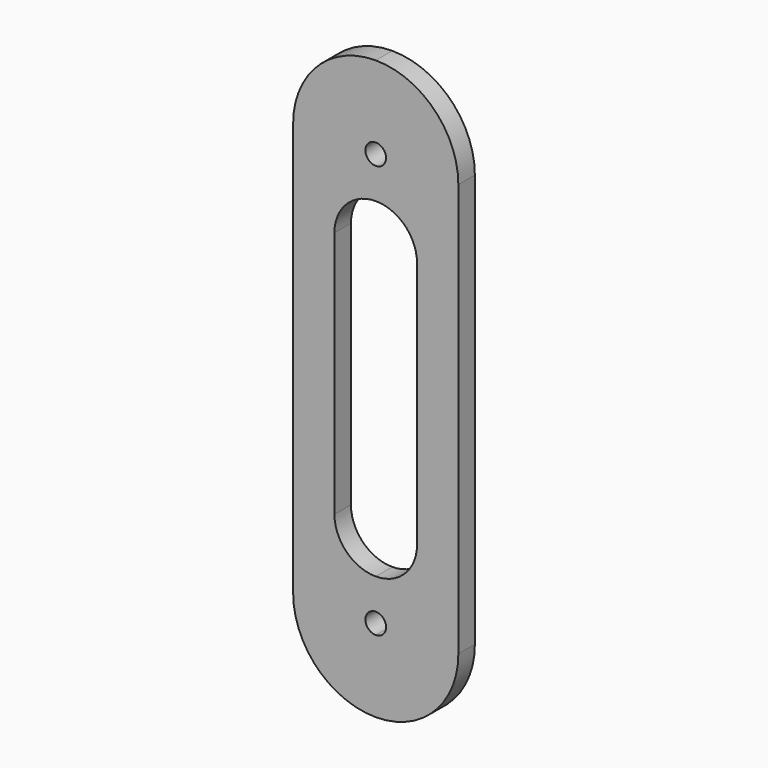
from build123d import *

# Parameters (mm, degrees)
F1_DEPTH = 1.5875


with BuildPart() as f1:
    # F0 (on Front) → F1 (new body, symmetric)
    with BuildSketch(Plane.XZ):
        with BuildLine():
            Line((0, 76.2), (0, 12.7))
            ThreePointArc((0, 12.7), (3.719744, 3.719744), (12.7, 0))
            Line((12.7, 0), (12.7, 11.1125))
            ThreePointArc((12.7, 11.1125), (11.1125, 12.7), (12.7, 14.2875))
            Line((12.7, 14.2875), (12.7, 19.05))
            ThreePointArc((12.7, 19.05), (8.209872, 20.909872), (6.35, 25.4))
            Line((6.35, 25.4), (6.35, 63.5))
            ThreePointArc((6.35, 63.5), (8.209872, 67.990128), (12.7, 69.85))
            Line((12.7, 69.85), (12.7, 74.6125))
            ThreePointArc((12.7, 74.6125), (11.1125, 76.2), (12.7, 77.7875))
            Line((12.7, 77.7875), (12.7, 88.9))
            ThreePointArc((12.7, 88.9), (3.719744, 85.180256), (0, 76.2))
        make_face()
        with BuildLine():
            Line((12.7, 11.1125), (12.7, 0))
            ThreePointArc((12.7, 0), (21.680256, 3.719744), (25.4, 12.7))
            Line((25.4, 12.7), (25.4, 76.2))
            ThreePointArc((25.4, 76.2), (21.680256, 85.180256), (12.7, 88.9))
            Line((12.7, 88.9), (12.7, 77.7875))
            ThreePointArc((12.7, 77.7875), (13.822532, 77.322532), (14.2875, 76.2))
            ThreePointArc((14.2875, 76.2), (13.822532, 75.077468), (12.7, 74.6125))
            Line((12.7, 74.6125), (12.7, 69.85))
            ThreePointArc((12.7, 69.85), (17.190128, 67.990128), (19.05, 63.5))
            Line((19.05, 63.5), (19.05, 25.4))
            ThreePointArc((19.05, 25.4), (17.190128, 20.909872), (12.7, 19.05))
            Line((12.7, 19.05), (12.7, 14.2875))
            ThreePointArc((12.7, 14.2875), (13.822532, 13.822532), (14.2875, 12.7))
            ThreePointArc((14.2875, 12.7), (13.822532, 11.577468), (12.7, 11.1125))
        make_face()
    extrude(amount=F1_DEPTH, both=True)


solid = f1.part
